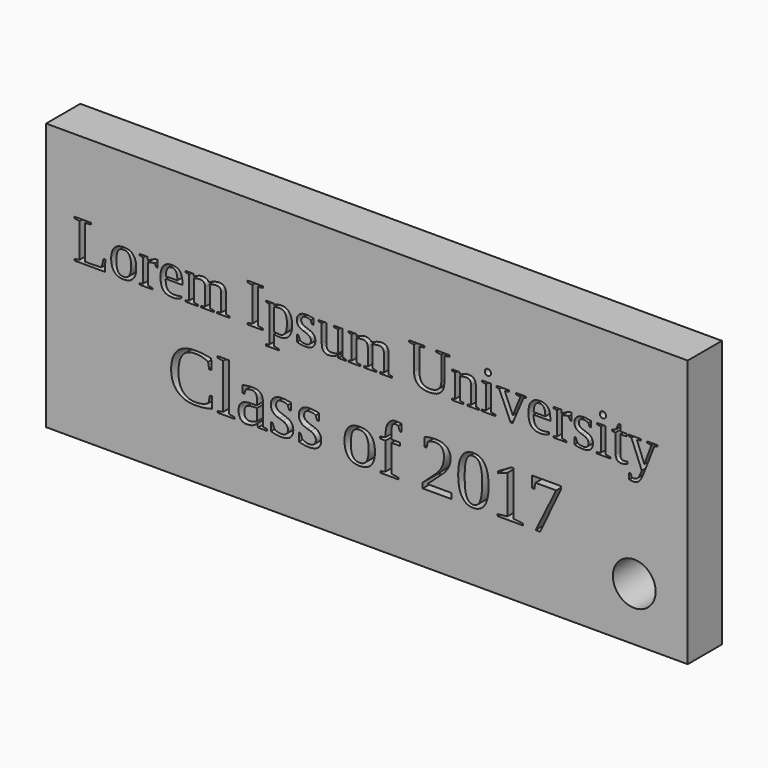
from build123d import *

# Parameters (mm, degrees)
F0_W           = 38.1
F0_H           = 15.875
F1_DEPTH       = 2.54
F2_TEXT_SIZE   = 3.5115391262
F2_TEXT_SIZE_2 = 4.2639789172
F3_DEPTH       = 1.27
F4_D           = 2.54


# Not quite as in the source:
# - Text() gives the source's letters only with a copy of the font that has no kerning and outlines rounded to 1/6400 em; it was checked with that copy


with BuildPart() as f1:
    # F0 (on Front) → F1 (new body)
    with BuildSketch(Plane.XZ):
        with Locations((19.05, -7.9375)):
            Rectangle(F0_W, F0_H)
    extrude(amount=F1_DEPTH)

    # F2 (on face) → F3 (cut)
    with BuildSketch(Plane.XZ.offset(2.54)):
        with Locations((1.5875, -6.6180420553)):
            Text('Lorem Ipsum University', F2_TEXT_SIZE, font='Tinos', text_align=(TextAlign.LEFT, TextAlign.BOTTOM))
        with Locations((7.2517702103, -11.8025359698)):
            Text('Class of 2017', F2_TEXT_SIZE_2, font='Tinos', text_align=(TextAlign.LEFT, TextAlign.BOTTOM))
    extrude(amount=-F3_DEPTH, mode=Mode.SUBTRACT)

    # F4 (through all)
    with Locations(Plane(origin=(0, 0, 0), x_dir=(1, 0, 0), z_dir=(0, 1, 0))):
        with Locations((34.925, 12.7)):
            Hole(F4_D / 2)


solid = f1.part
